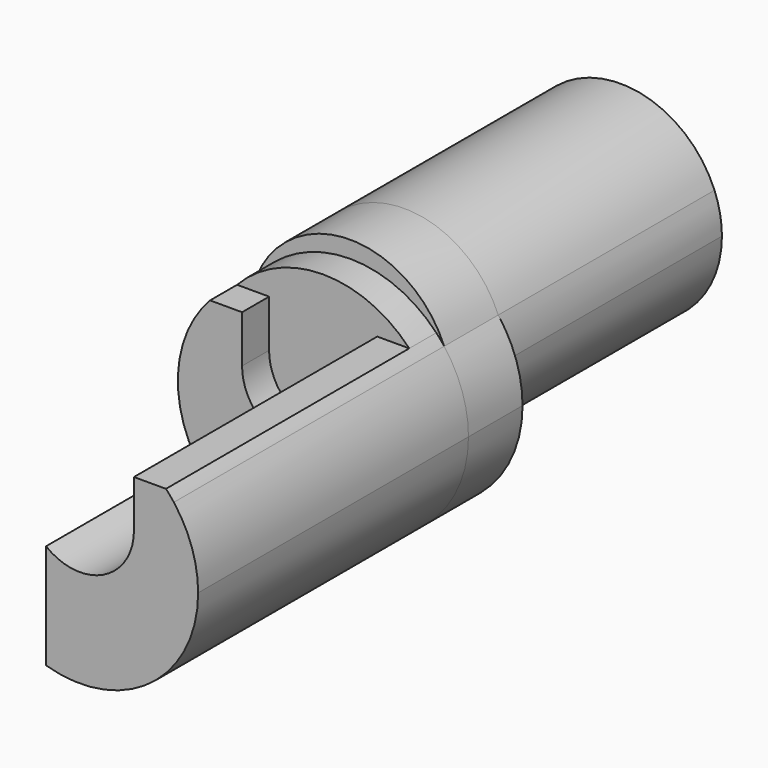
from build123d import *
from build123d import SkipClean  # not in build123d's __all__

# Parameters (mm, degrees)
F1_DEPTH = 50
F2_DEPTH = 10
F3_DEPTH = 5
F5_DEPTH = 50
F6_DEPTH = 10


# Not quite as in the source:
# - a feature of the source that left no trace in its solid (it failed there, or was rolled back) is left out


with BuildPart() as f1:
    # F0 (on Front) → F1 (new body)
    with BuildSketch(Plane.XZ):
        with BuildLine():
            ThreePointArc((-5, -14.1421356237), (8.6602540378, -12.2474487139), (15, 0))
            ThreePointArc((15, 0), (14.7238001625, 2.8652589369), (13.9053721633, 5.625))
            ThreePointArc((13.9053721633, 5.625), (13.3392841662, 6.3275548082), (12.7377392029, 7))
            Line((12.7377392029, 7), (8, 7))
            Line((8, 7), (8, 0))
            ThreePointArc((8, 0), (3.4641016151, -7.2111025509), (-5, -6.2449979984))
            Line((-5, -6.2449979984), (-5, -14.1421356237))
        make_face()
        with BuildLine():
            ThreePointArc((13.9053721633, 5.625), (14.7238001625, 2.8652589369), (15, 0))
            ThreePointArc((15, 0), (8.6602540378, -12.2474487139), (-5, -14.1421356237))
            Line((-5, -14.1421356237), (-5, -21.7705098312))
            ThreePointArc((-5, -21.7705098312), (10.4582503317, -19.0312152004), (17.5, -5))
            ThreePointArc((17.5, -5), (16.5770023354, 0.6082968512), (13.9053721633, 5.625))
        make_face()
    extrude(amount=F1_DEPTH)

    # F0 (on Front) → F2 (join)
    with BuildSketch(Plane.XZ):
        with BuildLine():
            Line((-5, -21.7705098312), (-5, -14.1421356237))
            ThreePointArc((-5, -14.1421356237), (-13.6761905094, -6.1613158619), (-13.9053721633, 5.625))
            ThreePointArc((-13.9053721633, 5.625), (-16.6427691172, -10.4100125798), (-5, -21.7705098312))
        make_face()
        with BuildLine():
            ThreePointArc((-13.9053721633, 5.625), (-13.6761905094, -6.1613158619), (-5, -14.1421356237))
            Line((-5, -14.1421356237), (-5, -6.2449979984))
            ThreePointArc((-5, -6.2449979984), (-7.2111025509, -3.4641016151), (-8, 0))
            Line((-8, 0), (-8, 7))
            Line((-8, 7), (-12.7377392029, 7))
            ThreePointArc((-12.7377392029, 7), (-13.3392841662, 6.3275548082), (-13.9053721633, 5.625))
        make_face()
    extrude(amount=F2_DEPTH)

    # F0 (on Front) → F3 (join)
    with BuildSketch(Plane.XZ):
        with BuildLine():
            ThreePointArc((13.9053721633, 5.625), (14.7238001625, 2.8652589369), (15, 0))
            ThreePointArc((15, 0), (8.6602540378, -12.2474487139), (-5, -14.1421356237))
            Line((-5, -14.1421356237), (-5, -21.7705098312))
            ThreePointArc((-5, -21.7705098312), (10.4582503317, -19.0312152004), (17.5, -5))
            ThreePointArc((17.5, -5), (16.5770023354, 0.6082968512), (13.9053721633, 5.625))
        make_face()
        with BuildLine():
            Line((-5, -21.7705098312), (-5, -14.1421356237))
            ThreePointArc((-5, -14.1421356237), (-13.6761905094, -6.1613158619), (-13.9053721633, 5.625))
            ThreePointArc((-13.9053721633, 5.625), (-16.6427691172, -10.4100125798), (-5, -21.7705098312))
        make_face()
        with BuildLine():
            Line((8, 7), (12.7377392029, 7))
            ThreePointArc((12.7377392029, 7), (0, 12.5), (-12.7377392029, 7))
            Line((-12.7377392029, 7), (-8, 7))
            Line((-8, 7), (-8, 0))
            ThreePointArc((-8, 0), (-7.2111025509, -3.4641016151), (-5, -6.2449979984))
            ThreePointArc((-5, -6.2449979984), (3.4641016151, -7.2111025509), (8, 0))
            Line((8, 0), (8, 7))
        make_face()
    extrude(amount=F3_DEPTH)

    # F0 (on Front) → F5 (join)
    with BuildSketch(Plane.XZ):
        with BuildLine():
            ThreePointArc((12.7377392029, 7), (13.3392841662, 6.3275548082), (13.9053721633, 5.625))
            ThreePointArc((13.9053721633, 5.625), (0, 15), (-13.9053721633, 5.625))
            ThreePointArc((-13.9053721633, 5.625), (-13.3392841662, 6.3275548082), (-12.7377392029, 7))
            ThreePointArc((-12.7377392029, 7), (0, 12.5), (12.7377392029, 7))
        make_face()
        with BuildLine():
            Line((8, 7), (12.7377392029, 7))
            ThreePointArc((12.7377392029, 7), (0, 12.5), (-12.7377392029, 7))
            Line((-12.7377392029, 7), (-8, 7))
            Line((-8, 7), (-8, 0))
            ThreePointArc((-8, 0), (-7.2111025509, -3.4641016151), (-5, -6.2449979984))
            ThreePointArc((-5, -6.2449979984), (3.4641016151, -7.2111025509), (8, 0))
            Line((8, 0), (8, 7))
        make_face()
        with BuildLine():
            ThreePointArc((-5, -14.1421356237), (8.6602540378, -12.2474487139), (15, 0))
            ThreePointArc((15, 0), (14.7238001625, 2.8652589369), (13.9053721633, 5.625))
            ThreePointArc((13.9053721633, 5.625), (13.3392841662, 6.3275548082), (12.7377392029, 7))
            Line((12.7377392029, 7), (8, 7))
            Line((8, 7), (8, 0))
            ThreePointArc((8, 0), (3.4641016151, -7.2111025509), (-5, -6.2449979984))
            Line((-5, -6.2449979984), (-5, -14.1421356237))
        make_face()
        with BuildLine():
            ThreePointArc((-13.9053721633, 5.625), (-13.6761905094, -6.1613158619), (-5, -14.1421356237))
            Line((-5, -14.1421356237), (-5, -6.2449979984))
            ThreePointArc((-5, -6.2449979984), (-7.2111025509, -3.4641016151), (-8, 0))
            Line((-8, 0), (-8, 7))
            Line((-8, 7), (-12.7377392029, 7))
            ThreePointArc((-12.7377392029, 7), (-13.3392841662, 6.3275548082), (-13.9053721633, 5.625))
        make_face()
    extrude(amount=-F5_DEPTH)

    # F0 (on Front) → F6 (join)
    with BuildSketch(Plane.XZ):
        with BuildLine():
            ThreePointArc((-5, -14.1421356237), (8.6602540378, -12.2474487139), (15, 0))
            ThreePointArc((15, 0), (14.7238001625, 2.8652589369), (13.9053721633, 5.625))
            ThreePointArc((13.9053721633, 5.625), (13.3392841662, 6.3275548082), (12.7377392029, 7))
            Line((12.7377392029, 7), (8, 7))
            Line((8, 7), (8, 0))
            ThreePointArc((8, 0), (3.4641016151, -7.2111025509), (-5, -6.2449979984))
            Line((-5, -6.2449979984), (-5, -14.1421356237))
        make_face()
        with BuildLine():
            ThreePointArc((13.9053721633, 5.625), (14.7238001625, 2.8652589369), (15, 0))
            ThreePointArc((15, 0), (8.6602540378, -12.2474487139), (-5, -14.1421356237))
            Line((-5, -14.1421356237), (-5, -21.7705098312))
            ThreePointArc((-5, -21.7705098312), (10.4582503317, -19.0312152004), (17.5, -5))
            ThreePointArc((17.5, -5), (16.5770023354, 0.6082968512), (13.9053721633, 5.625))
        make_face()
        with BuildLine():
            ThreePointArc((12.7377392029, 7), (13.3392841662, 6.3275548082), (13.9053721633, 5.625))
            ThreePointArc((13.9053721633, 5.625), (0, 15), (-13.9053721633, 5.625))
            ThreePointArc((-13.9053721633, 5.625), (-13.3392841662, 6.3275548082), (-12.7377392029, 7))
            ThreePointArc((-12.7377392029, 7), (0, 12.5), (12.7377392029, 7))
        make_face()
        with BuildLine():
            Line((-5, -21.7705098312), (-5, -14.1421356237))
            ThreePointArc((-5, -14.1421356237), (-13.6761905094, -6.1613158619), (-13.9053721633, 5.625))
            ThreePointArc((-13.9053721633, 5.625), (-16.6427691172, -10.4100125798), (-5, -21.7705098312))
        make_face()
        with BuildLine():
            ThreePointArc((-13.9053721633, 5.625), (-13.6761905094, -6.1613158619), (-5, -14.1421356237))
            Line((-5, -14.1421356237), (-5, -6.2449979984))
            ThreePointArc((-5, -6.2449979984), (-7.2111025509, -3.4641016151), (-8, 0))
            Line((-8, 0), (-8, 7))
            Line((-8, 7), (-12.7377392029, 7))
            ThreePointArc((-12.7377392029, 7), (-13.3392841662, 6.3275548082), (-13.9053721633, 5.625))
        make_face()
    with SkipClean():  # cleaning this boolean's faces spoils the solid; the shape is the same uncleaned
        extrude(amount=-F6_DEPTH)


solid = f1.part
